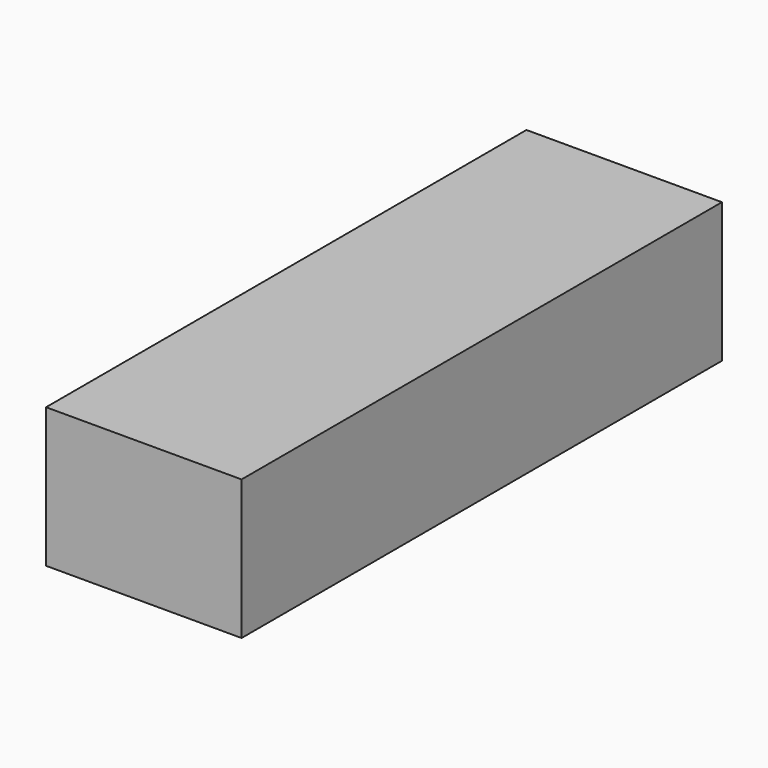
from build123d import *

# Parameters (mm, degrees)
F0_W     = 35.56
F0_H     = 109.22
F1_DEPTH = 25.4


# Not quite as in the source:
# - the program builds the solid bodies; features that only make, move or delete a surface that nothing else refers to are left out


with BuildPart() as f1:
    # F0 (on Top) → F1 (new body)
    with BuildSketch(Plane.XY):
        Rectangle(F0_W, F0_H)
    extrude(amount=F1_DEPTH)


solid = f1.part
